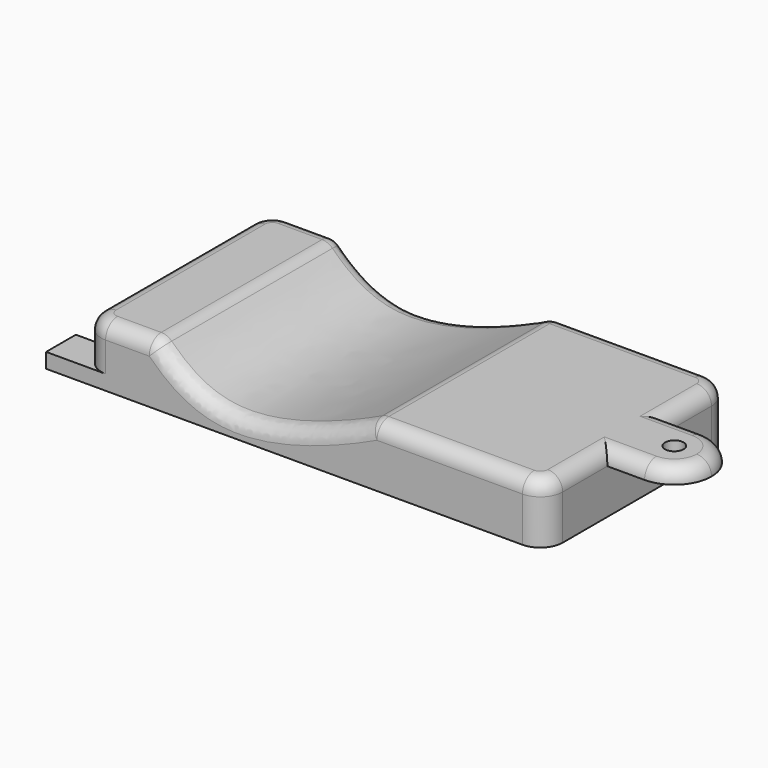
from build123d import *

# Parameters (mm, degrees)
F0_W     = 5
F0_H     = 5
F1_DEPTH = 2
F0_R     = 1.25
F2_DEPTH = 8
F3_DEPTH = 6
F5_R     = 3
F6_DEPTH = 50
F7_R     = 1.99999


# Not quite as in the source:
# - a fillet or chamfer is up to 0.001 mm smaller than in the source, because OpenCascade refuses the exact size


with BuildPart() as f1:
    # F0 (on Top) → F1 (new body)
    with BuildSketch(Plane.XY):
        with Locations((-33.5, 13)):
            Rectangle(F0_W, F0_H)
        with BuildLine():
            Line((-31, -15.5), (28, -15.5))
            ThreePointArc((28, -15.5), (30.1213203436, -14.6213203436), (31, -12.5))
            Line((31, -12.5), (31, -5))
            Line((31, -5), (31, 5))
            Line((31, 5), (31, 12.5))
            ThreePointArc((31, 12.5), (30.1213203436, 14.6213203436), (28, 15.5))
            Line((28, 15.5), (-31, 15.5))
            Line((-31, 15.5), (-31, 10.5))
            Line((-31, 10.5), (-31, -10.5))
            Line((-31, -10.5), (-31, -15.5))
        make_face()
        with Locations((-33.5, -13)):
            Rectangle(F0_W, F0_H)
    extrude(amount=F1_DEPTH)

    # F0 (on Top) → F2 (join)
    with BuildSketch(Plane.XY):
        with BuildLine():
            Line((31, 5), (31, -5))
            Line((31, -5), (36, -5))
            ThreePointArc((36, -5), (39.5355339059, -3.5355339059), (41, 0))
            ThreePointArc((41, 0), (39.5355339059, 3.5355339059), (36, 5))
            Line((36, 5), (31, 5))
        make_face()
        with Locations((36, 0)):
            Circle(F0_R, mode=Mode.SUBTRACT)
        with BuildLine():
            Line((-31, -15.5), (28, -15.5))
            ThreePointArc((28, -15.5), (30.1213203436, -14.6213203436), (31, -12.5))
            Line((31, -12.5), (31, -5))
            Line((31, -5), (31, 5))
            Line((31, 5), (31, 12.5))
            ThreePointArc((31, 12.5), (30.1213203436, 14.6213203436), (28, 15.5))
            Line((28, 15.5), (-31, 15.5))
            Line((-31, 15.5), (-31, 10.5))
            Line((-31, 10.5), (-31, -10.5))
            Line((-31, -10.5), (-31, -15.5))
        make_face()
    extrude(amount=F2_DEPTH)

    # F0 (on Top) → F3 (cut)
    with BuildSketch(Plane.XY):
        with BuildLine():
            Line((31, 5), (31, -5))
            Line((31, -5), (36, -5))
            ThreePointArc((36, -5), (39.5355339059, -3.5355339059), (41, 0))
            ThreePointArc((41, 0), (39.5355339059, 3.5355339059), (36, 5))
            Line((36, 5), (31, 5))
        make_face()
        with Locations((36, 0)):
            Circle(F0_R, mode=Mode.SUBTRACT)
    extrude(amount=F3_DEPTH, mode=Mode.SUBTRACT)

    # F5
    f5_edges = [f1.edges().sort_by_distance(p)[0] for p in [
        (-31, 15.5, 5),
        (-31, -15.5, 5),
    ]]
    fillet(f5_edges, radius=F5_R)

    # F4 (on face) → F6 (cut)
    with BuildSketch(Plane.XZ.offset(15.5)):
        with BuildLine():
            Line((8, 8), (-21.3, 8))
            add(Edge.make_bspline(
                [(-21.3, 8), (-18.6027030945, 5.1925020669), (-11.9176320955, 0.5356481102), (0.5768376855, 4.4751283983), (8, 8)],
                knots=[0, 0, 0, 0, 0.4179419715, 1, 1, 1, 1], degree=3))
        make_face()
    extrude(amount=-F6_DEPTH, mode=Mode.SUBTRACT)

    # F7 (radius 2 in the source; OpenCascade refuses exactly that, so slightly less here)
    f7_edges = [f1.edges().sort_by_distance(p)[0] for p in [
        (33.5, -5, 8),
        (30.12132, -14.62132, 8),
        (-7.010651, -15.5, 2.945097),
        (8, 0, 8),
        (-7.010651, 15.5, 2.945097),
        (-21.3, 0, 8),
        (33.5, 5, 8),
        (31, 8.75, 8),
        (30.12132, 14.62132, 8),
        (-24.65, -15.5, 8),
        (-30.12132, -14.62132, 8),
        (-31, 0, 8),
        (-30.12132, 14.62132, 8),
        (-24.65, 15.5, 8),
        (18, -15.5, 8),
        (31, -8.75, 8),
        (41, 0, 8),
        (18, 15.5, 8),
    ]]
    fillet(f7_edges, radius=F7_R)


solid = f1.part
